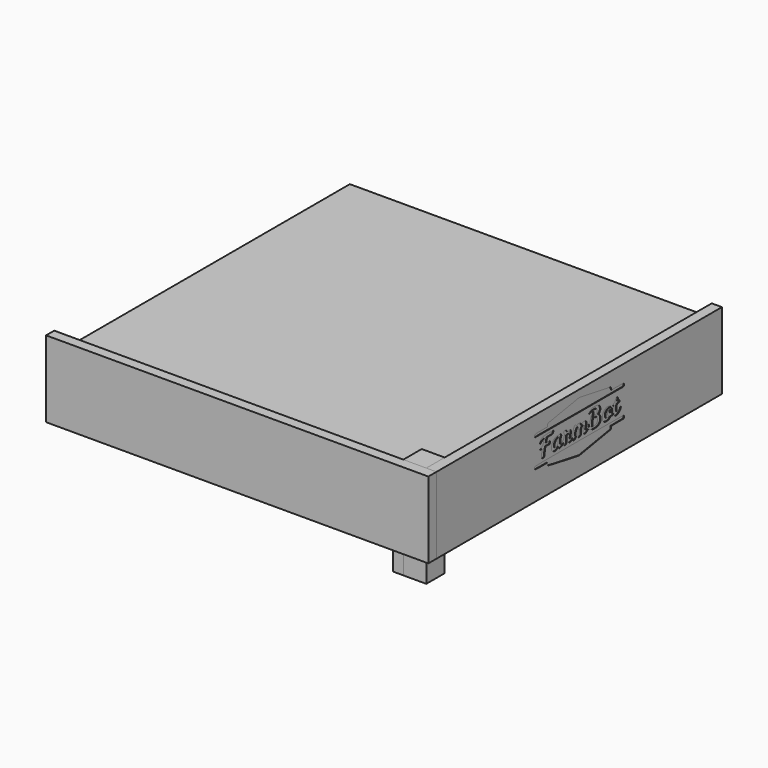
from build123d import *

# Parameters (mm, degrees)
F0_W      = 1420
F0_H      = 1400
F1_DEPTH  = 250
F2_W      = 1400
F2_H      = 300
F3_DEPTH  = 40
F4_W      = 1500
F4_H      = 300
F5_DEPTH  = 40
F8_DEPTH  = 2
F9_W      = 90
F9_H      = 90
F10_DEPTH = 400
F11_W     = 1310
F11_H     = 100
F11_W_2   = 90
F12_DEPTH = 40


# Not quite as in the source:
# - ends of sketch curves that miss each other by under 0.0002 mm in the source are joined


with BuildPart() as f1:
    # F0 (on Top) → F1 (new body)
    with BuildSketch(Plane.XY):
        Rectangle(F0_W, F0_H)
    extrude(amount=F1_DEPTH)


with BuildPart() as f3:
    # F2 (on face) → F3 (new body)
    with BuildSketch(Plane.YZ.offset(710)):
        with Locations((0, 150)):
            Rectangle(F2_W, F2_H)
    extrude(amount=F3_DEPTH)

    # F7 (on face) → F8 (cut)
    with BuildSketch(Plane.YZ.offset(750)):
        with BuildLine():
            add(Edge.make_bspline(
                [(-4.016334356, 72.8065287048), (-5.8572942886, 73.1809385763), (-39.5929322315, 78.9888205837), (-78.984412348, 85.7129139551)],
                knots=[0, 0, 0, 0, 1, 1, 1, 1], degree=3))
            Line((-4.016334356, 72.8065287048), (-4.016334356, 72.8068259994))
            add(Edge.make_bspline(
                [(-0.3005735092, 72.0381908331), (-0.5032862592, 72.0863905113), (-2.1753744233, 72.4324751651), (-4.016334356, 72.8068259994)],
                knots=[0, 0, 0, 0, 1, 1, 1, 1], degree=3))
            add(Edge.make_bspline(
                [(151.2723663775, 98.4387001135), (148.676128451, 97.484108227), (0.916521078, 71.7478014768), (-0.3005735092, 72.0381908331)],
                knots=[0, 0, 0, 0, 1, 1, 1, 1], degree=3))
            add(Edge.make_bspline(
                [(156.8864966424, 107.1581420894), (156.682750741, 102.4686106916), (154.961366493, 99.7950150225), (151.2723663775, 98.4387001135)],
                knots=[0, 0, 0, 0, 1, 1, 1, 1], degree=3))
            Line((156.8864966424, 107.1581420894), (157.0211584469, 110.2570841054))
            Line((157.0211584469, 110.2570841054), (187.0264111787, 110.6289954372))
            Line((187.0264111787, 110.6289954372), (217.031661802, 111.0009046605))
            Line((217.031661802, 111.0009046605), (218.4528986835, 112.756920567))
            add(Edge.make_bspline(
                [(219.1460210206, 120.2694054908), (220.3090628104, 118.0961355543), (219.991895855, 114.6584273921), (218.4528986835, 112.756920567)],
                knots=[0, 0, 0, 0, 1, 1, 1, 1], degree=3))
            add(Edge.make_bspline(
                [(216.0597551404, 122.4519590311), (217.3567418541, 121.9998350852), (218.7455483222, 121.0176917904), (219.1460210206, 120.2694054908)],
                knots=[0, 0, 0, 0, 1, 1, 1, 1], degree=3))
            add(Edge.make_bspline(
                [(0.1496528115, 123.2728421426), (154.1515528614, 123.2734367318), (214.3591393453, 123.0447560362), (216.0597551404, 122.4519590311)],
                knots=[0, 0, 0, 0, 1, 1, 1, 1], degree=3))
            add(Edge.make_bspline(
                [(-215.9613637404, 121.9711514272), (-213.5426612954, 123.2003634051), (-201.6878745281, 123.2717710387), (0.1496528115, 123.2728421426)],
                knots=[0, 0, 0, 0, 1, 1, 1, 1], degree=3))
            add(Edge.make_bspline(
                [(-218.848203979, 114.5822018992), (-220.2410081107, 117.4869746952), (-219.1152651971, 120.3683645327), (-215.9613637404, 121.9711514272)],
                knots=[0, 0, 0, 0, 1, 1, 1, 1], degree=3))
            add(Edge.make_bspline(
                [(-185.4265998016, 110.6400037714), (-216.4088891081, 110.6519039894), (-216.996895664, 110.7211694151), (-218.848203979, 114.5822018992)],
                knots=[0, 0, 0, 0, 1, 1, 1, 1], degree=3))
            Line((-185.4265998016, 110.6400037714), (-156.7071019511, 110.6286960341))
            Line((-156.7071019511, 110.6286960341), (-156.2651745776, 106.897328275))
            add(Edge.make_bspline(
                [(-152.1331190558, 99.0087066408), (-154.6528194356, 100.7735886736), (-155.7990841107, 102.96197214), (-156.2651745776, 106.897328275)],
                knots=[0, 0, 0, 0, 1, 1, 1, 1], degree=3))
            add(Edge.make_bspline(
                [(-78.984412348, 85.7129139551), (-121.5139044734, 92.9726794898), (-151.2258750247, 98.3732446974), (-152.1331190558, 99.0087066408)],
                knots=[0, 0, 0, 0, 1, 1, 1, 1], degree=3))
        make_face()
        with BuildLine():
            add(Edge.make_bspline(
                [(65.159129077, 135.442487088), (57.7102272459, 137.1835054306), (51.0152265762, 139.7460035824), (47.1901772814, 142.3200456204)],
                knots=[0, 0, 0, 0, 1, 1, 1, 1], degree=3))
            add(Edge.make_bspline(
                [(90.2559171831, 136.6657468485), (84.4646963243, 134.649334605), (71.2983701672, 134.0075641123), (65.159129077, 135.442487088)],
                knots=[0, 0, 0, 0, 1, 1, 1, 1], degree=3))
            add(Edge.make_bspline(
                [(103.986993446, 148.1080278656), (101.6414549919, 143.5165868191), (95.6912932695, 138.5582083271), (90.2559171831, 136.6657468485)],
                knots=[0, 0, 0, 0, 1, 1, 1, 1], degree=3))
            add(Edge.make_bspline(
                [(103.8137128617, 166.0933877931), (106.0736831818, 161.4249643121), (106.1609781546, 152.3636251085), (103.986993446, 148.1080278656)],
                knots=[0, 0, 0, 0, 1, 1, 1, 1], degree=3))
            add(Edge.make_bspline(
                [(94.823104472, 175.3412698722), (96.2922416287, 175.3412698722), (102.3565939974, 169.1034049872), (103.8137128617, 166.0933877931)],
                knots=[0, 0, 0, 0, 1, 1, 1, 1], degree=3))
            add(Edge.make_bspline(
                [(98.2033883894, 179.2463356931), (96.0013778661, 177.0985466452), (94.4802921673, 175.3412698722), (94.823104472, 175.3412698722)],
                knots=[0, 0, 0, 0, 1, 1, 1, 1], degree=3))
            add(Edge.make_bspline(
                [(102.9736700618, 196.7100848596), (104.880235112, 189.1385458418), (103.6217469953, 184.5313650491), (98.2033883894, 179.2463356931)],
                knots=[0, 0, 0, 0, 1, 1, 1, 1], degree=3))
            add(Edge.make_bspline(
                [(90.8209835596, 208.7957029643), (96.6539774728, 206.6194389971), (101.756122153, 201.5454403145), (102.9736700618, 196.7100848596)],
                knots=[0, 0, 0, 0, 1, 1, 1, 1], degree=3))
            add(Edge.make_bspline(
                [(66.2443429349, 209.9609860602), (72.3511177676, 211.7240716746), (84.5184286341, 211.1471683342), (90.8209835596, 208.7957029643)],
                knots=[0, 0, 0, 0, 1, 1, 1, 1], degree=3))
            add(Edge.make_bspline(
                [(47.3073978025, 196.1849044547), (47.3073978025, 200.1826039005), (57.1330266109, 207.3304622645), (66.2443429349, 209.9609860602)],
                knots=[0, 0, 0, 0, 1, 1, 1, 1], degree=3))
            add(Edge.make_bspline(
                [(55.8823335165, 197.1655191071), (49.815482608, 194.2584586186), (47.3073978025, 193.9716410144), (47.3073978025, 196.1849044547)],
                knots=[0, 0, 0, 0, 1, 1, 1, 1], degree=3))
            add(Edge.make_bspline(
                [(74.7146625756, 201.2201409813), (67.9096650112, 201.6238522933), (62.9647596576, 200.5592108003), (55.8823335165, 197.1655191071)],
                knots=[0, 0, 0, 0, 1, 1, 1, 1], degree=3))
            add(Edge.make_bspline(
                [(87.8011261251, 189.8458033777), (87.811240467, 197.6464679787), (84.358062443, 200.6480407409), (74.7146625756, 201.2201409813)],
                knots=[0, 0, 0, 0, 1, 1, 1, 1], degree=3))
            add(Edge.make_bspline(
                [(86.6978278997, 183.1514036226), (87.3013949816, 184.3787095415), (87.7979128132, 187.3911894313), (87.8011261251, 189.8458033777)],
                knots=[0, 0, 0, 0, 1, 1, 1, 1], degree=3))
            add(Edge.make_bspline(
                [(79.7417814836, 180.5045497085), (85.3421687256, 180.9016319833), (85.6487427158, 181.0182811084), (86.6978278997, 183.1514036226)],
                knots=[0, 0, 0, 0, 1, 1, 1, 1], degree=3))
            add(Edge.make_bspline(
                [(72.5653554275, 178.4617520418), (73.6520557584, 179.8037799421), (74.9105375497, 180.1620051798), (79.7417814836, 180.5045497085)],
                knots=[0, 0, 0, 0, 1, 1, 1, 1], degree=3))
            add(Edge.make_bspline(
                [(71.6432487748, 175.3212288424), (71.4178530791, 176.18315126), (71.8146970966, 177.53473054), (72.5653554275, 178.4617520418)],
                knots=[0, 0, 0, 0, 1, 1, 1, 1], degree=3))
            add(Edge.make_bspline(
                [(80.1404113772, 171.6221586629), (74.7976604817, 171.6221586629), (72.3296113495, 172.6965708168), (71.6432487748, 175.3212288424)],
                knots=[0, 0, 0, 0, 1, 1, 1, 1], degree=3))
            add(Edge.make_bspline(
                [(86.7987499294, 168.9074815182), (85.1384797529, 171.5938397705), (85.0690372156, 171.6221586629), (80.1404113772, 171.6221586629)],
                knots=[0, 0, 0, 0, 1, 1, 1, 1], degree=3))
            add(Edge.make_bspline(
                [(88.2208786948, 152.2906424461), (89.6927547571, 155.8441436936), (88.8602687221, 165.5719140827), (86.7987499294, 168.9074815182)],
                knots=[0, 0, 0, 0, 1, 1, 1, 1], degree=3))
            add(Edge.make_bspline(
                [(73.3411741592, 144.1226524407), (80.2797139293, 144.0946856633), (86.163823538, 147.3244330878), (88.2208786948, 152.2906424461)],
                knots=[0, 0, 0, 0, 1, 1, 1, 1], degree=3))
            add(Edge.make_bspline(
                [(64.0859967658, 145.7092968707), (64.5914692795, 145.1092952156), (70.2740911606, 144.1350903192), (73.3411741592, 144.1226524407)],
                knots=[0, 0, 0, 0, 1, 1, 1, 1], degree=3))
            add(Edge.make_bspline(
                [(67.2581365084, 173.10980399), (65.380075896, 164.0625261886), (63.355693627, 146.5761826323), (64.0859967658, 145.7092968707)],
                knots=[0, 0, 0, 0, 1, 1, 1, 1], degree=3))
            add(Edge.make_bspline(
                [(64.1258595443, 194.0137408821), (71.0929206201, 200.2917784911), (71.8507688418, 195.2341162524), (67.2581365084, 173.10980399)],
                knots=[0, 0, 0, 0, 1, 1, 1, 1], degree=3))
            add(Edge.make_bspline(
                [(51.2455666395, 156.1878478821), (52.1745469122, 169.1434153588), (59.1016503282, 189.4864121548), (64.1258595443, 194.0137408821)],
                knots=[0, 0, 0, 0, 1, 1, 1, 1], degree=3))
            add(Edge.make_bspline(
                [(49.1270115609, 150.0513140705), (50.6979773904, 150.0513140705), (50.8337398174, 150.4445589257), (51.2455666395, 156.1878478821)],
                knots=[0, 0, 0, 0, 1, 1, 1, 1], degree=3))
            add(Edge.make_bspline(
                [(47.8439007039, 154.4122189657), (47.4678483324, 150.2650604564), (47.5307398461, 150.0513140705), (49.1270115609, 150.0513140705)],
                knots=[0, 0, 0, 0, 1, 1, 1, 1], degree=3))
            add(Edge.make_bspline(
                [(47.346225321, 159.3250945156), (47.9544521269, 158.9491897371), (48.1131947942, 157.3820760866), (47.8439007039, 154.4122189657)],
                knots=[0, 0, 0, 0, 1, 1, 1, 1], degree=3))
            add(Edge.make_bspline(
                [(40.2767367663, 153.8484619505), (44.1420768595, 157.6213181203), (46.7872924906, 159.6705360853), (47.346225321, 159.3250945156)],
                knots=[0, 0, 0, 0, 1, 1, 1, 1], degree=3))
            add(Edge.make_bspline(
                [(31.6871303016, 148.8881921588), (31.6871303016, 146.5425988845), (34.3922033547, 148.1047028046), (40.2767367663, 153.8484619505)],
                knots=[0, 0, 0, 0, 1, 1, 1, 1], degree=3))
            add(Edge.make_bspline(
                [(33.5457276056, 157.6281010759), (32.5235022511, 153.4087505814), (31.6871303016, 149.4757875625), (31.6871303016, 148.8881921588)],
                knots=[0, 0, 0, 0, 1, 1, 1, 1], degree=3))
            add(Edge.make_bspline(
                [(34.454660523, 175.3189369329), (35.9054708379, 172.4517581991), (35.5739894637, 166.000016203), (33.5457276056, 157.6281010759)],
                knots=[0, 0, 0, 0, 1, 1, 1, 1], degree=3))
            add(Edge.make_bspline(
                [(31.008432024, 178.8520935306), (32.3925492495, 177.9193390924), (33.9433517578, 176.3294223132), (34.454660523, 175.3189369329)],
                knots=[0, 0, 0, 0, 1, 1, 1, 1], degree=3))
            add(Edge.make_bspline(
                [(12.2549598312, 175.6194237633), (17.328709714, 180.4677631911), (26.3128725037, 182.0164319254), (31.008432024, 178.8520935306)],
                knots=[0, 0, 0, 0, 1, 1, 1, 1], degree=3))
            Line((12.2549598312, 175.6194237633), (10.3026177375, 173.7538094634))
            Line((10.3026177375, 173.7538094634), (9.803917637, 175.7407431547))
            add(Edge.make_bspline(
                [(3.7036305738, 182.8231397772), (7.1800945665, 181.1402203906), (8.9704258608, 179.061641948), (9.803917637, 175.7407431547)],
                knots=[0, 0, 0, 0, 1, 1, 1, 1], degree=3))
            add(Edge.make_bspline(
                [(-9.3102298383, 181.1432144214), (-4.897680021, 184.339650091), (-0.5803214055, 184.8969678316), (3.7036305738, 182.8231397772)],
                knots=[0, 0, 0, 0, 1, 1, 1, 1], degree=3))
            add(Edge.make_bspline(
                [(-12.8048372357, 179.7640183703), (-12.5960499768, 179.1376481597), (-11.4597625929, 179.5860970383), (-9.3102298383, 181.1432144214)],
                knots=[0, 0, 0, 0, 1, 1, 1, 1], degree=3))
            add(Edge.make_bspline(
                [(-15.3708333431, 183.2623219198), (-14.129697954, 181.8487430098), (-12.9749951724, 180.2745069397), (-12.8048372357, 179.7640183703)],
                knots=[0, 0, 0, 0, 1, 1, 1, 1], degree=3))
            add(Edge.make_bspline(
                [(-19.8929204082, 185.6076579604), (-18.0910916141, 185.7864437661), (-17.1655987548, 185.3064458155), (-15.3708333431, 183.2623219198)],
                knots=[0, 0, 0, 0, 1, 1, 1, 1], degree=3))
            add(Edge.make_bspline(
                [(-24.5291833602, 181.4253596507), (-22.5975654413, 184.6497937249), (-21.7387551289, 185.4245055086), (-19.8929204082, 185.6076579604)],
                knots=[0, 0, 0, 0, 1, 1, 1, 1], degree=3))
            add(Edge.make_bspline(
                [(-30.5734946991, 162.8976711126), (-30.0157046607, 168.8709395837), (-27.5831853963, 176.3273328171), (-24.5291833602, 181.4253596507)],
                knots=[0, 0, 0, 0, 1, 1, 1, 1], degree=3))
            Line((-30.5734946991, 162.8976711126), (-31.0145744668, 158.1742523469))
            Line((-31.0145744668, 158.1742523469), (-36.5582754293, 152.9970523761))
            add(Edge.make_bspline(
                [(-41.9533185479, 161.2011921402), (-46.2177292053, 145.6912968422), (-45.5189877894, 144.6287490622), (-36.5582754293, 152.9970523761)],
                knots=[0, 0, 0, 0, 1, 1, 1, 1], degree=3))
            Line((-41.9533185479, 161.2011921402), (-38.8598163906, 172.4524371272))
            Line((-38.8598163906, 172.4524371272), (-40.591500526, 175.8997008862))
            add(Edge.make_bspline(
                [(-49.5751214383, 178.7903975207), (-43.8279824112, 181.0896170539), (-43.0772102228, 180.8480346158), (-40.591500526, 175.8997008862)],
                knots=[0, 0, 0, 0, 1, 1, 1, 1], degree=3))
            add(Edge.make_bspline(
                [(-56.7338089163, 176.8289130908), (-55.4931437165, 176.8289130908), (-52.2717395171, 177.711580768), (-49.5751214383, 178.7903975207)],
                knots=[0, 0, 0, 0, 1, 1, 1, 1], degree=3))
            add(Edge.make_bspline(
                [(-60.4027342665, 179.9901583567), (-59.1897090308, 177.2766408719), (-58.6700865591, 176.8289130908), (-56.7338089163, 176.8289130908)],
                knots=[0, 0, 0, 0, 1, 1, 1, 1], degree=3))
            add(Edge.make_bspline(
                [(-69.0367072066, 187.2424240552), (-65.3745247511, 187.2424240552), (-62.6046435831, 184.9158091406), (-60.4027342665, 179.9901583567)],
                knots=[0, 0, 0, 0, 1, 1, 1, 1], degree=3))
            add(Edge.make_bspline(
                [(-75.8335745017, 182.4645223637), (-75.2378382861, 185.6400462044), (-72.9583519458, 187.2424240552), (-69.0367072066, 187.2424240552)],
                knots=[0, 0, 0, 0, 1, 1, 1, 1], degree=3))
            add(Edge.make_bspline(
                [(-73.1293047766, 174.9538338584), (-75.504376603, 177.570779092), (-76.3243910239, 179.8482307565), (-75.8335745017, 182.4645223637)],
                knots=[0, 0, 0, 0, 1, 1, 1, 1], degree=3))
            add(Edge.make_bspline(
                [(-73.5941575702, 168.4115540589), (-71.8157560126, 173.3110218331), (-71.8028732464, 173.4923293716), (-73.1293047766, 174.9538338584)],
                knots=[0, 0, 0, 0, 1, 1, 1, 1], degree=3))
            add(Edge.make_bspline(
                [(-75.4232657797, 161.7355359659), (-75.4232657797, 162.635834689), (-74.6001750976, 165.6400430417), (-73.5941575702, 168.4115540589)],
                knots=[0, 0, 0, 0, 1, 1, 1, 1], degree=3))
            add(Edge.make_bspline(
                [(-88.836580498, 148.1839771486), (-86.1418073325, 149.0392642036), (-75.4232657797, 159.868274949), (-75.4232657797, 161.7355359659)],
                knots=[0, 0, 0, 0, 1, 1, 1, 1], degree=3))
            add(Edge.make_bspline(
                [(-91.7759638679, 158.4052354944), (-91.7634669522, 148.8162784919), (-91.3520259805, 147.385604088), (-88.836580498, 148.1839771486)],
                knots=[0, 0, 0, 0, 1, 1, 1, 1], degree=3))
            add(Edge.make_bspline(
                [(-89.3916991019, 171.9891952065), (-91.6808380287, 167.347055942), (-91.7868478022, 166.7431009012), (-91.7759638679, 158.4052354944)],
                knots=[0, 0, 0, 0, 1, 1, 1, 1], degree=3))
            Line((-89.3916991019, 171.9891952065), (-86.9960443683, 176.8473305969))
            Line((-86.9960443683, 176.8473305969), (-88.4025641127, 179.4590742292))
            add(Edge.make_bspline(
                [(-99.2536505637, 183.8698149772), (-96.484471517, 186.3758946255), (-90.9064657091, 184.1085467606), (-88.4025641127, 179.4590742292)],
                knots=[0, 0, 0, 0, 1, 1, 1, 1], degree=3))
            add(Edge.make_bspline(
                [(-103.995105202, 183.5086758307), (-101.1316584643, 182.8669643753), (-100.2910442684, 182.9309923556), (-99.2536505637, 183.8698149772)],
                knots=[0, 0, 0, 0, 1, 1, 1, 1], degree=3))
            add(Edge.make_bspline(
                [(-125.3558046793, 177.0251928916), (-119.2897381225, 182.5055216088), (-110.8922472257, 185.0543610766), (-103.995105202, 183.5086758307)],
                knots=[0, 0, 0, 0, 1, 1, 1, 1], degree=3))
            add(Edge.make_bspline(
                [(-136.1680172253, 154.0805098765), (-135.3619398067, 163.6033451856), (-131.7662838712, 171.2337105823), (-125.3558046793, 177.0251928916)],
                knots=[0, 0, 0, 0, 1, 1, 1, 1], degree=3))
            add(Edge.make_bspline(
                [(-132.8503781303, 141.000683798), (-135.7783251461, 144.4803421264), (-136.6798067222, 148.034450614), (-136.1680172253, 154.0805098765)],
                knots=[0, 0, 0, 0, 1, 1, 1, 1], degree=3))
            add(Edge.make_bspline(
                [(-105.2882671467, 142.3403354499), (-111.8650542049, 134.3615639714), (-126.6588743356, 133.6424968818), (-132.8503781303, 141.000683798)],
                knots=[0, 0, 0, 0, 1, 1, 1, 1], degree=3))
            Line((-105.2882671467, 142.3403354499), (-103.1712596868, 144.9086065991))
            Line((-103.1712596868, 144.9086065991), (-101.8746777999, 141.5135633751))
            add(Edge.make_bspline(
                [(-92.8607475974, 136.6719942521), (-97.5893089271, 135.612316103), (-100.1452665976, 136.9851740862), (-101.8746777999, 141.5135633751)],
                knots=[0, 0, 0, 0, 1, 1, 1, 1], degree=3))
            add(Edge.make_bspline(
                [(-80.2807517606, 143.4154876777), (-84.0660626767, 139.9263053796), (-88.1801308207, 137.72096347), (-92.8607475974, 136.6719942521)],
                knots=[0, 0, 0, 0, 1, 1, 1, 1], degree=3))
            Line((-80.2807517606, 143.4154876777), (-77.1040830193, 146.3436118051))
            Line((-77.1040830193, 146.3436118051), (-76.5911127779, 142.4328678681))
            add(Edge.make_bspline(
                [(-71.278158814, 135.1748882095), (-74.5421098772, 135.1748882095), (-75.8785903866, 137.0005849107), (-76.5911127779, 142.4328678681)],
                knots=[0, 0, 0, 0, 1, 1, 1, 1], degree=3))
            add(Edge.make_bspline(
                [(-63.5888742655, 138.7692158074), (-64.6134400243, 136.8547966976), (-68.2072974329, 135.1748882095), (-71.278158814, 135.1748882095)],
                knots=[0, 0, 0, 0, 1, 1, 1, 1], degree=3))
            add(Edge.make_bspline(
                [(-63.2356735175, 148.2452620063), (-63.0271582516, 143.638930928), (-63.1801532232, 139.5328538942), (-63.5888742655, 138.7692158074)],
                knots=[0, 0, 0, 0, 1, 1, 1, 1], degree=3))
            add(Edge.make_bspline(
                [(-62.2461927389, 161.952470362), (-63.3001527109, 157.6209681139), (-63.5213609805, 154.5565860684), (-63.2356735175, 148.2452620063)],
                knots=[0, 0, 0, 0, 1, 1, 1, 1], degree=3))
            Line((-62.2461927389, 161.952470362), (-60.8887708819, 167.5311361218))
            Line((-60.8887708819, 167.5311361218), (-56.5878773271, 167.7553658322))
            Line((-56.5878773271, 167.7553658322), (-52.2869795554, 167.9796081935))
            Line((-52.2869795554, 167.9796081935), (-53.4416464929, 165.7467359603))
            add(Edge.make_bspline(
                [(-55.4287825976, 142.2411992963), (-57.7602723003, 147.3184471348), (-56.7418780401, 159.3647780739), (-53.4416464929, 165.7467359603)],
                knots=[0, 0, 0, 0, 1, 1, 1, 1], degree=3))
            add(Edge.make_bspline(
                [(-46.8226056486, 136.4516441308), (-51.4490958312, 136.343285519), (-53.2887695957, 137.580885), (-55.4287825976, 142.2411992963)],
                knots=[0, 0, 0, 0, 1, 1, 1, 1], degree=3))
            add(Edge.make_bspline(
                [(-34.7589746937, 142.046140301), (-38.9331279746, 138.0212289109), (-42.0781380033, 136.5626826109), (-46.8226056486, 136.4516441308)],
                knots=[0, 0, 0, 0, 1, 1, 1, 1], degree=3))
            Line((-34.7589746937, 142.046140301), (-31.6577070326, 145.0366035224))
            Line((-31.6577070326, 145.0366035224), (-31.1348290796, 141.4074039001))
            add(Edge.make_bspline(
                [(-20.9866082165, 137.1811270738), (-27.4172422958, 133.6811156617), (-30.1879035987, 134.8349919221), (-31.1348290796, 141.4074039001)],
                knots=[0, 0, 0, 0, 1, 1, 1, 1], degree=3))
            add(Edge.make_bspline(
                [(-17.0202975988, 146.4728695949), (-15.6770741947, 140.7752754515), (-16.0687166108, 139.8577547261), (-20.9866082165, 137.1811270738)],
                knots=[0, 0, 0, 0, 1, 1, 1, 1], degree=3))
            add(Edge.make_bspline(
                [(-15.6596750807, 163.0891857658), (-18.4834382601, 157.2065984742), (-18.7585981205, 153.8462607053), (-17.0202975988, 146.4728695949)],
                knots=[0, 0, 0, 0, 1, 1, 1, 1], degree=3))
            add(Edge.make_bspline(
                [(-6.9396743596, 173.10980399), (-9.6736672196, 173.10980399), (-12.2962062304, 170.0961096201), (-15.6596750807, 163.0891857658)],
                knots=[0, 0, 0, 0, 1, 1, 1, 1], degree=3))
            add(Edge.make_bspline(
                [(-4.7272015965, 161.2086476985), (-3.788897659, 171.7136305194), (-4.0484442816, 173.10980399), (-6.9396743596, 173.10980399)],
                knots=[0, 0, 0, 0, 1, 1, 1, 1], degree=3))
            add(Edge.make_bspline(
                [(-4.525977428, 137.4063562001), (-5.6931834507, 139.6765610451), (-5.7759557502, 149.4673009613), (-4.7272015965, 161.2086476985)],
                knots=[0, 0, 0, 0, 1, 1, 1, 1], degree=3))
            add(Edge.make_bspline(
                [(5.8697823076, 137.8887683516), (1.6427970346, 134.9062203355), (-3.1267698657, 134.6848581474), (-4.525977428, 137.4063562001)],
                knots=[0, 0, 0, 0, 1, 1, 1, 1], degree=3))
            add(Edge.make_bspline(
                [(8.9170983778, 143.0290552967), (8.9921768617, 140.3920584909), (8.6863049928, 139.8760836764), (5.8697823076, 137.8887683516)],
                knots=[0, 0, 0, 0, 1, 1, 1, 1], degree=3))
            add(Edge.make_bspline(
                [(8.0994285781, 149.8588843402), (8.5032410968, 147.7146543936), (8.8711948259, 144.6412459779), (8.9170983778, 143.0290552967)],
                knots=[0, 0, 0, 0, 1, 1, 1, 1], degree=3))
            add(Edge.make_bspline(
                [(11.8364618026, 164.3851203518), (8.2937453912, 158.3399276714), (7.2594089715, 154.3193365411), (8.0994285781, 149.8588843402)],
                knots=[0, 0, 0, 0, 1, 1, 1, 1], degree=3))
            add(Edge.make_bspline(
                [(19.4445322125, 169.5121492227), (16.9706088762, 170.6393427653), (14.5429222304, 169.0033389973), (11.8364618026, 164.3851203518)],
                knots=[0, 0, 0, 0, 1, 1, 1, 1], degree=3))
            add(Edge.make_bspline(
                [(20.0972751953, 156.9236604592), (21.7406923522, 167.0442729852), (21.6651921738, 168.5003481556), (19.4445322125, 169.5121492227)],
                knots=[0, 0, 0, 0, 1, 1, 1, 1], degree=3))
            add(Edge.make_bspline(
                [(29.9765772762, 136.6959169795), (21.0318534621, 134.6913459169), (17.6211084445, 141.6748235584), (20.0972751953, 156.9236604592)],
                knots=[0, 0, 0, 0, 1, 1, 1, 1], degree=3))
            add(Edge.make_bspline(
                [(40.5706114274, 142.2913640708), (37.0579491812, 139.1179191838), (34.311765134, 137.6674673092), (29.9765772762, 136.6959169795)],
                knots=[0, 0, 0, 0, 1, 1, 1, 1], degree=3))
            Line((40.5706114274, 142.2913640708), (43.414653894, 144.8608222899))
            Line((43.414653894, 144.8608222899), (47.1901772814, 142.3200456204))
        make_face()
        with BuildLine():
            add(Edge.make_bspline(
                [(-112.8487493354, 147.12334597), (-107.2523681908, 149.2378063953), (-103.7298952226, 155.255928399), (-103.704842354, 162.7456397128)],
                knots=[0, 0, 0, 0, 1, 1, 1, 1], degree=3))
            add(Edge.make_bspline(
                [(-119.8084497341, 148.2519079112), (-117.7226771838, 146.1661290354), (-116.0850730852, 145.9005795921), (-112.8487493354, 147.12334597)],
                knots=[0, 0, 0, 0, 1, 1, 1, 1], degree=3))
            add(Edge.make_bspline(
                [(-121.3827300822, 155.5541422963), (-121.7050311677, 150.5320626372), (-121.5995970072, 150.0430488588), (-119.8084497341, 148.2519079112)],
                knots=[0, 0, 0, 0, 1, 1, 1, 1], degree=3))
            add(Edge.make_bspline(
                [(-113.1935857735, 171.6807657607), (-118.2073812447, 167.7155684164), (-120.9487010461, 162.3171622844), (-121.3827300822, 155.5541422963)],
                knots=[0, 0, 0, 0, 1, 1, 1, 1], degree=3))
            add(Edge.make_bspline(
                [(-102.5050330232, 176.6371981327), (-103.2842548293, 177.4164199387), (-109.707190876, 174.4380066369), (-113.1935857735, 171.6807657607)],
                knots=[0, 0, 0, 0, 1, 1, 1, 1], degree=3))
            add(Edge.make_bspline(
                [(-102.8935232732, 171.9302739463), (-102.4562914675, 174.2955160746), (-102.281465373, 176.4136410249), (-102.5050330232, 176.6371981327)],
                knots=[0, 0, 0, 0, 1, 1, 1, 1], degree=3))
            add(Edge.make_bspline(
                [(-103.704842354, 162.7456397128), (-103.6958581533, 165.4319452533), (-103.3307656211, 169.5650254926), (-102.8935232732, 171.9302739463)],
                knots=[0, 0, 0, 0, 1, 1, 1, 1], degree=3))
        make_face(mode=Mode.SUBTRACT)
        with BuildLine():
            add(Edge.make_bspline(
                [(-183.8353504679, 136.0044582271), (-185.9055983362, 138.132147208), (-184.3907473902, 157.7927010795), (-181.4402903235, 167.0887638605)],
                knots=[0, 0, 0, 0, 1, 1, 1, 1], degree=3))
            add(Edge.make_bspline(
                [(-172.6445933361, 136.8661023264), (-175.0771821801, 135.2721815582), (-182.5621051531, 134.6959276273), (-183.8353504679, 136.0044582271)],
                knots=[0, 0, 0, 0, 1, 1, 1, 1], degree=3))
            add(Edge.make_bspline(
                [(-170.2903005048, 143.1477116875), (-170.6883337007, 138.8356242529), (-171.0299800201, 137.924055745), (-172.6445933361, 136.8661023264)],
                knots=[0, 0, 0, 0, 1, 1, 1, 1], degree=3))
            add(Edge.make_bspline(
                [(-166.7193158044, 164.4668742592), (-168.5288805836, 156.9223995927), (-169.6202237706, 150.4069754058), (-170.2903005048, 143.1477116875)],
                knots=[0, 0, 0, 0, 1, 1, 1, 1], degree=3))
            Line((-166.7193158044, 164.4668742592), (-165.1349822601, 171.0723006975))
            Line((-165.1349822601, 171.0723006975), (-155.7366206169, 170.561396759))
            add(Edge.make_bspline(
                [(-145.4061033417, 171.1736865911), (-146.1904972305, 170.2285512032), (-147.8281203053, 170.1314918948), (-155.7366206169, 170.561396759)],
                knots=[0, 0, 0, 0, 1, 1, 1, 1], degree=3))
            add(Edge.make_bspline(
                [(-143.0245458543, 179.6641969631), (-142.4149274567, 178.6778008795), (-144.067318272, 172.7868176509), (-145.4061033417, 171.1736865911)],
                knots=[0, 0, 0, 0, 1, 1, 1, 1], degree=3))
            add(Edge.make_bspline(
                [(-152.8097404882, 180.7098390117), (-146.9706699576, 180.5774733336), (-143.3498578384, 180.190556004), (-143.0245458543, 179.6641969631)],
                knots=[0, 0, 0, 0, 1, 1, 1, 1], degree=3))
            add(Edge.make_bspline(
                [(-161.8077032295, 182.0356822781), (-162.0354920413, 181.0973340627), (-160.6049019763, 180.8865416466), (-152.8097404882, 180.7098390117)],
                knots=[0, 0, 0, 0, 1, 1, 1, 1], degree=3))
            add(Edge.make_bspline(
                [(-159.5762373473, 191.135941773), (-160.6545839107, 186.7444555947), (-161.6587438739, 182.6493341833), (-161.8077032295, 182.0356822781)],
                knots=[0, 0, 0, 0, 1, 1, 1, 1], degree=3))
            Line((-159.5762373473, 191.135941773), (-157.615617391, 199.1204735981))
            Line((-157.615617391, 199.1204735981), (-144.4951715925, 199.1320174843))
            add(Edge.make_bspline(
                [(-127.1451787271, 204.8682029974), (-129.5670712908, 199.1924821463), (-129.7105507267, 199.1450436265), (-144.4951715925, 199.1320174843)],
                knots=[0, 0, 0, 0, 1, 1, 1, 1], degree=3))
            add(Edge.make_bspline(
                [(-143.6058980714, 210.4809711891), (-124.5845022954, 210.0475599355), (-124.8905639268, 210.151922992), (-127.1451787271, 204.8682029974)],
                knots=[0, 0, 0, 0, 1, 1, 1, 1], degree=3))
            add(Edge.make_bspline(
                [(-178.2221289546, 208.0834652168), (-170.9524198642, 210.3288512335), (-162.5302345391, 210.9121685468), (-143.6058980714, 210.4809711891)],
                knots=[0, 0, 0, 0, 1, 1, 1, 1], degree=3))
            add(Edge.make_bspline(
                [(-193.6909933804, 194.2595655665), (-193.6909933804, 199.5125271664), (-187.2047567764, 205.3090149891), (-178.2221289546, 208.0834652168)],
                knots=[0, 0, 0, 0, 1, 1, 1, 1], degree=3))
            add(Edge.make_bspline(
                [(-187.2104454348, 192.5154625289), (-191.9760441901, 188.1226880739), (-193.6909933804, 188.5842326743), (-193.6909933804, 194.2595655665)],
                knots=[0, 0, 0, 0, 1, 1, 1, 1], degree=3))
            add(Edge.make_bspline(
                [(-174.4256473519, 198.7819815533), (-179.2901208102, 197.9940475394), (-183.5117505634, 195.9247927616), (-187.2104454348, 192.5154625289)],
                knots=[0, 0, 0, 0, 1, 1, 1, 1], degree=3))
            add(Edge.make_bspline(
                [(-171.7383192023, 197.926180031), (-171.2007620647, 199.1979198965), (-171.4222655204, 199.2684588394), (-174.4256473519, 198.7819815533)],
                knots=[0, 0, 0, 0, 1, 1, 1, 1], degree=3))
            add(Edge.make_bspline(
                [(-175.4829829882, 187.6204056789), (-173.7456333875, 192.5262937514), (-172.060531732, 197.1638871495), (-171.7383192023, 197.926180031)],
                knots=[0, 0, 0, 0, 1, 1, 1, 1], degree=3))
            Line((-175.4829829882, 187.6204056789), (-178.6418056193, 178.7006082251))
            Line((-178.6418056193, 178.7006082251), (-182.9551349441, 177.0298715918))
            add(Edge.make_bspline(
                [(-191.4595274982, 169.9953541597), (-191.4595274982, 172.0848523807), (-187.7059448742, 175.1896791431), (-182.9551349441, 177.0298715918)],
                knots=[0, 0, 0, 0, 1, 1, 1, 1], degree=3))
            add(Edge.make_bspline(
                [(-186.2026441398, 168.6468701171), (-190.7828090761, 168.6468701171), (-191.4595274982, 168.8204669722), (-191.4595274982, 169.9953541597)],
                knots=[0, 0, 0, 0, 1, 1, 1, 1], degree=3))
            add(Edge.make_bspline(
                [(-181.4402903235, 167.0887638605), (-180.9701579151, 168.5700247333), (-181.2050227602, 168.6468701171), (-186.2026441398, 168.6468701171)],
                knots=[0, 0, 0, 0, 1, 1, 1, 1], degree=3))
        make_face()
        with BuildLine():
            add(Edge.make_bspline(
                [(126.8915395812, 136.5790464649), (121.0492641726, 138.4646659507), (115.6936241857, 143.4566640345), (114.2137759893, 148.3958765127)],
                knots=[0, 0, 0, 0, 1, 1, 1, 1], degree=3))
            add(Edge.make_bspline(
                [(135.0784046312, 136.1378106702), (131.6010065852, 136.0495647764), (127.916944512, 136.248075341), (126.8915395812, 136.5790464649)],
                knots=[0, 0, 0, 0, 1, 1, 1, 1], degree=3))
            add(Edge.make_bspline(
                [(150.8902205209, 142.1234980436), (146.205388908, 137.8323582819), (142.2070780052, 136.3187682024), (135.0784046312, 136.1378106702)],
                knots=[0, 0, 0, 0, 1, 1, 1, 1], degree=3))
            add(Edge.make_bspline(
                [(159.0409632224, 144.5494283319), (153.8801460818, 144.6225606958), (153.4926447054, 144.5071787627), (150.8902205209, 142.1234980436)],
                knots=[0, 0, 0, 0, 1, 1, 1, 1], degree=3))
            add(Edge.make_bspline(
                [(167.1898040818, 146.170514658), (164.955063742, 144.7809069703), (163.4756920604, 144.4865916385), (159.0409632224, 144.5494283319)],
                knots=[0, 0, 0, 0, 1, 1, 1, 1], degree=3))
            add(Edge.make_bspline(
                [(171.1089144372, 144.472667287), (170.2890433924, 147.9068163479), (170.1081448975, 147.9852093504), (167.1898040818, 146.170514658)],
                knots=[0, 0, 0, 0, 1, 1, 1, 1], degree=3))
            add(Edge.make_bspline(
                [(177.3418454968, 136.7062695788), (174.417255169, 137.4856769305), (172.0824277546, 140.3949745082), (171.1089144372, 144.472667287)],
                knots=[0, 0, 0, 0, 1, 1, 1, 1], degree=3))
            add(Edge.make_bspline(
                [(203.2722603214, 153.1740649564), (199.9971828495, 143.6680889923), (185.578516881, 134.5111621941), (177.3418454968, 136.7062695788)],
                knots=[0, 0, 0, 0, 1, 1, 1, 1], degree=3))
            add(Edge.make_bspline(
                [(202.5944307343, 159.7210044798), (203.9272403934, 159.7210044798), (204.297070663, 156.1486281877), (203.2722603214, 153.1740649564)],
                knots=[0, 0, 0, 0, 1, 1, 1, 1], degree=3))
            add(Edge.make_bspline(
                [(197.2628926949, 155.4440252186), (199.7803433347, 157.7963613875), (202.1794981324, 159.7210044798), (202.5944307343, 159.7210044798)],
                knots=[0, 0, 0, 0, 1, 1, 1, 1], degree=3))
            add(Edge.make_bspline(
                [(184.7096133114, 148.0247389902), (186.5054371762, 147.3356206422), (192.1652116508, 150.6806888541), (197.2628926949, 155.4440252186)],
                knots=[0, 0, 0, 0, 1, 1, 1, 1], degree=3))
            add(Edge.make_bspline(
                [(183.3629383381, 164.4379902963), (182.363301048, 154.7271783504), (182.8548175831, 148.7364875722), (184.7096133114, 148.0247389902)],
                knots=[0, 0, 0, 0, 1, 1, 1, 1], degree=3))
            add(Edge.make_bspline(
                [(184.671648158, 174.2936353172), (184.4505242274, 173.7174277727), (183.8615962691, 169.2823910977), (183.3629383381, 164.4379902963)],
                knots=[0, 0, 0, 0, 1, 1, 1, 1], degree=3))
            add(Edge.make_bspline(
                [(190.4999422863, 175.3412698722), (186.5194817106, 175.3412698722), (184.9665580791, 175.0621271075), (184.671648158, 174.2936353172)],
                knots=[0, 0, 0, 0, 1, 1, 1, 1], degree=3))
            add(Edge.make_bspline(
                [(196.7428717219, 177.6837257396), (195.9275823876, 175.345018736), (195.9175861201, 175.3412698722), (190.4999422863, 175.3412698722)],
                knots=[0, 0, 0, 0, 1, 1, 1, 1], degree=3))
            add(Edge.make_bspline(
                [(197.5594683091, 181.7747482807), (197.5594683091, 180.8130466254), (197.1920206134, 178.9720866928), (196.7428717219, 177.6837257396)],
                knots=[0, 0, 0, 0, 1, 1, 1, 1], degree=3))
            add(Edge.make_bspline(
                [(192.3527138812, 183.5233128459), (197.3225772221, 183.5233128459), (197.5594683091, 183.4437538582), (197.5594683091, 181.7747482807)],
                knots=[0, 0, 0, 0, 1, 1, 1, 1], degree=3))
            add(Edge.make_bspline(
                [(187.154943654, 184.0811808978), (187.1489935449, 183.7743517825), (189.488997259, 183.5233128459), (192.3527138812, 183.5233128459)],
                knots=[0, 0, 0, 0, 1, 1, 1, 1], degree=3))
            add(Edge.make_bspline(
                [(189.0151539393, 187.8774221347), (187.9969494416, 186.0963132985), (187.159822659, 184.3880036877), (187.154943654, 184.0811808978)],
                knots=[0, 0, 0, 0, 1, 1, 1, 1], degree=3))
            Line((189.0151539393, 187.8774221347), (190.8664369526, 191.1158037535))
            Line((190.8664369526, 191.1158037535), (189.4216378924, 194.3819687127))
            add(Edge.make_bspline(
                [(175.8766954614, 187.8002921071), (180.2222823048, 199.6004715487), (185.8941341092, 202.3565105957), (189.4216378924, 194.3819687127)],
                knots=[0, 0, 0, 0, 1, 1, 1, 1], degree=3))
            add(Edge.make_bspline(
                [(171.6049536455, 183.5233128459), (174.2094019634, 183.5233128459), (174.3555486168, 183.6696323941), (175.8766954614, 187.8002921071)],
                knots=[0, 0, 0, 0, 1, 1, 1, 1], degree=3))
            add(Edge.make_bspline(
                [(166.6589518863, 178.0362201494), (167.4597222799, 182.3046347959), (168.5581984289, 183.5233128459), (171.6049536455, 183.5233128459)],
                knots=[0, 0, 0, 0, 1, 1, 1, 1], degree=3))
            add(Edge.make_bspline(
                [(168.7155326367, 175.3412698722), (166.1736237176, 175.3412698722), (166.157377938, 175.3625717685), (166.6589518863, 178.0362201494)],
                knots=[0, 0, 0, 0, 1, 1, 1, 1], degree=3))
            add(Edge.make_bspline(
                [(171.6558901208, 174.96313433), (171.4479188408, 175.1711119355), (170.1247470089, 175.3412698722), (168.7155326367, 175.3412698722)],
                knots=[0, 0, 0, 0, 1, 1, 1, 1], degree=3))
            add(Edge.make_bspline(
                [(171.0633925188, 169.5704231819), (171.5972176604, 172.3284378675), (171.8638635094, 174.7551609414), (171.6558901208, 174.96313433)],
                knots=[0, 0, 0, 0, 1, 1, 1, 1], degree=3))
            add(Edge.make_bspline(
                [(170.0653597763, 161.8961720414), (170.0802371573, 163.3589964319), (170.5295062316, 166.8124148217), (171.0633925188, 169.5704231819)],
                knots=[0, 0, 0, 0, 1, 1, 1, 1], degree=3))
            add(Edge.make_bspline(
                [(164.3103793405, 154.9731632788), (168.4131819167, 157.046128968), (170.0356071227, 158.9977752658), (170.0653597763, 161.8961720414)],
                knots=[0, 0, 0, 0, 1, 1, 1, 1], degree=3))
            add(Edge.make_bspline(
                [(159.9969825446, 155.4440252186), (159.3218897547, 153.3744794716), (160.8220910347, 153.2107144231), (164.3103793405, 154.9731632788)],
                knots=[0, 0, 0, 0, 1, 1, 1, 1], degree=3))
            add(Edge.make_bspline(
                [(160.8654117079, 162.6962930256), (160.6880238195, 159.6280250655), (160.297250094, 156.3645020222), (159.9969825446, 155.4440252186)],
                knots=[0, 0, 0, 0, 1, 1, 1, 1], degree=3))
            add(Edge.make_bspline(
                [(159.662026408, 170.7109232936), (160.946280057, 168.6605983807), (161.1367573419, 167.3917914002), (160.8654117079, 162.6962930256)],
                knots=[0, 0, 0, 0, 1, 1, 1, 1], degree=3))
            add(Edge.make_bspline(
                [(151.3701931698, 174.5974472086), (155.578619669, 174.5974472086), (157.9129726772, 173.5032913194), (159.662026408, 170.7109232936)],
                knots=[0, 0, 0, 0, 1, 1, 1, 1], degree=3))
            add(Edge.make_bspline(
                [(143.0223061938, 150.7450267799), (134.4666840867, 160.2150553987), (139.5002190761, 174.5974472086), (151.3701931698, 174.5974472086)],
                knots=[0, 0, 0, 0, 1, 1, 1, 1], degree=3))
            Line((143.0223061938, 150.7450267799), (145.5799232321, 147.9140694928))
            Line((145.5799232321, 147.9140694928), (142.7465559611, 147.1272845964))
            add(Edge.make_bspline(
                [(128.0949860269, 157.8614478209), (127.974663943, 148.8059954722), (133.6963241899, 144.6141120471), (142.7465559611, 147.1272845964)],
                knots=[0, 0, 0, 0, 1, 1, 1, 1], degree=3))
            add(Edge.make_bspline(
                [(139.4740951035, 175.1445915701), (132.6681234248, 172.3008759168), (128.1966797574, 165.5093810093), (128.0949860269, 157.8614478209)],
                knots=[0, 0, 0, 0, 1, 1, 1, 1], degree=3))
            add(Edge.make_bspline(
                [(147.8310864631, 176.6410060338), (144.689123177, 176.425648775), (140.9284771706, 175.7522575223), (139.4740951035, 175.1445915701)],
                knots=[0, 0, 0, 0, 1, 1, 1, 1], degree=3))
            add(Edge.make_bspline(
                [(154.4196851834, 179.4299646598), (155.8959046988, 177.6512847838), (154.60629553, 177.1053907465), (147.8310864631, 176.6410060338)],
                knots=[0, 0, 0, 0, 1, 1, 1, 1], degree=3))
            add(Edge.make_bspline(
                [(134.2487755763, 183.5381839015), (141.5169897598, 185.2174556309), (151.2640948404, 183.2322656462), (154.4196851834, 179.4299646598)],
                knots=[0, 0, 0, 0, 1, 1, 1, 1], degree=3))
            add(Edge.make_bspline(
                [(115.873689834, 168.0333299609), (119.5918480138, 176.0268712883), (126.3236162246, 181.7071380059), (134.2487755763, 183.5381839015)],
                knots=[0, 0, 0, 0, 1, 1, 1, 1], degree=3))
            add(Edge.make_bspline(
                [(114.2137759893, 148.3958765127), (112.7557062041, 153.2624542264), (113.5890841228, 163.1217595554), (115.873689834, 168.0333299609)],
                knots=[0, 0, 0, 0, 1, 1, 1, 1], degree=3))
        make_face()
        with BuildLine():
            add(Edge.make_bspline(
                [(154.1673811634, 161.807776446), (154.5451245298, 164.9969758385), (154.4085587748, 165.7218096), (153.353818668, 166.1265624973)],
                knots=[0, 0, 0, 0, 1, 1, 1, 1], degree=3))
            add(Edge.make_bspline(
                [(153.0188013856, 157.2806838676), (153.400888205, 157.6627580362), (153.9177549034, 159.6999450578), (154.1673811634, 161.807776446)],
                knots=[0, 0, 0, 0, 1, 1, 1, 1], degree=3))
            add(Edge.make_bspline(
                [(150.5547267238, 162.3445239303), (150.676058766, 159.1179371058), (152.044273893, 156.3061395072), (153.0188013856, 157.2806838676)],
                knots=[0, 0, 0, 0, 1, 1, 1, 1], degree=3))
            add(Edge.make_bspline(
                [(153.353818668, 166.1265624973), (151.5209215337, 166.8299088169), (150.4409514466, 165.3707131074), (150.5547267238, 162.3445239303)],
                knots=[0, 0, 0, 0, 1, 1, 1, 1], degree=3))
        make_face(mode=Mode.SUBTRACT)
        with BuildLine():
            add(Edge.make_bspline(
                [(-216.0056606363, 222.4186630898), (-220.5355954355, 224.7150446191), (-220.5109663698, 230.4882591239), (-215.9613869336, 232.8003803994)],
                knots=[0, 0, 0, 0, 1, 1, 1, 1], degree=3))
            add(Edge.make_bspline(
                [(1.4420831164, 221.6531084016), (-171.405891124, 221.5111344149), (-214.5147851296, 221.6629275574), (-216.0056606363, 222.4186630898)],
                knots=[0, 0, 0, 0, 1, 1, 1, 1], degree=3))
            Line((1.4420831164, 221.6531084016), (217.0302934034, 221.83019267))
            Line((217.0302934034, 221.83019267), (218.4522450571, 223.5861959257))
            add(Edge.make_bspline(
                [(219.1460210206, 231.098634463), (220.3093010677, 228.9250545811), (219.9918368178, 225.487529856), (218.4522450571, 223.5861959257)],
                knots=[0, 0, 0, 0, 1, 1, 1, 1], degree=3))
            add(Edge.make_bspline(
                [(185.6431394505, 234.1032581848), (214.5555688476, 234.1032581848), (217.6883687129, 233.8223021339), (219.1460210206, 231.098634463)],
                knots=[0, 0, 0, 0, 1, 1, 1, 1], degree=3))
            Line((185.6431394505, 234.1032581848), (157.5847383504, 234.1032581848))
            Line((157.5847383504, 234.1032581848), (157.0955411349, 237.7907655019))
            add(Edge.make_bspline(
                [(150.085998558, 246.7412391201), (153.8600924011, 245.6872011346), (156.4942364439, 242.3237027657), (157.0955411349, 237.7907655019)],
                knots=[0, 0, 0, 0, 1, 1, 1, 1], degree=3))
            add(Edge.make_bspline(
                [(0.7615336, 272.0381908331), (4.0187733957, 272.0381908331), (145.063651123, 248.1438792754), (150.085998558, 246.7412391201)],
                knots=[0, 0, 0, 0, 1, 1, 1, 1], degree=3))
            add(Edge.make_bspline(
                [(-151.8719721027, 245.7178288042), (-149.3783050312, 247.0073536341), (-4.2228423562, 272.0381908331), (0.7615336, 272.0381908331)],
                knots=[0, 0, 0, 0, 1, 1, 1, 1], degree=3))
            add(Edge.make_bspline(
                [(-156.4999086974, 236.3196695743), (-156.4999086974, 239.9977351521), (-154.3019422241, 244.461244638), (-151.8719721027, 245.7178288042)],
                knots=[0, 0, 0, 0, 1, 1, 1, 1], degree=3))
            Line((-156.4999086974, 236.3196695743), (-156.4999086974, 234.1032581848))
            Line((-156.4999086974, 234.1032581848), (-184.9511076565, 234.1020690064))
            add(Edge.make_bspline(
                [(-215.9613869336, 232.8003803994), (-213.6575329782, 233.9712024522), (-210.564789871, 234.101027421), (-184.9511076565, 234.1020690064)],
                knots=[0, 0, 0, 0, 1, 1, 1, 1], degree=3))
        make_face()
    extrude(amount=-F8_DEPTH, mode=Mode.SUBTRACT)


with BuildPart() as f5:
    # F4 (on face) → F5 (new body)
    with BuildSketch(Plane.XZ.offset(700)):
        with Locations((0, 150)):
            Rectangle(F4_W, F4_H)
    extrude(amount=F5_DEPTH)


with BuildPart() as f10:
    # F9 (on face) → F10 (new body)
    with BuildSketch(Plane.XY.offset(300)):
        with Locations((665, -655)):
            Rectangle(F9_W, F9_H)
    extrude(amount=-F10_DEPTH)


with BuildPart() as f12:
    # F11 (on face) → F12 (new body)
    with BuildSketch(Plane(origin=(620, 0, 0), x_dir=(0, -1, 0), z_dir=(-1, 0, 0))):
        with Locations((-45, -50)):
            Rectangle(F11_W, F11_H)
        with Locations((655, -50)):
            Rectangle(F11_W_2, F11_H)
    extrude(amount=F12_DEPTH)


solid = Compound([f1.part, f3.part, f5.part, f10.part, f12.part])
